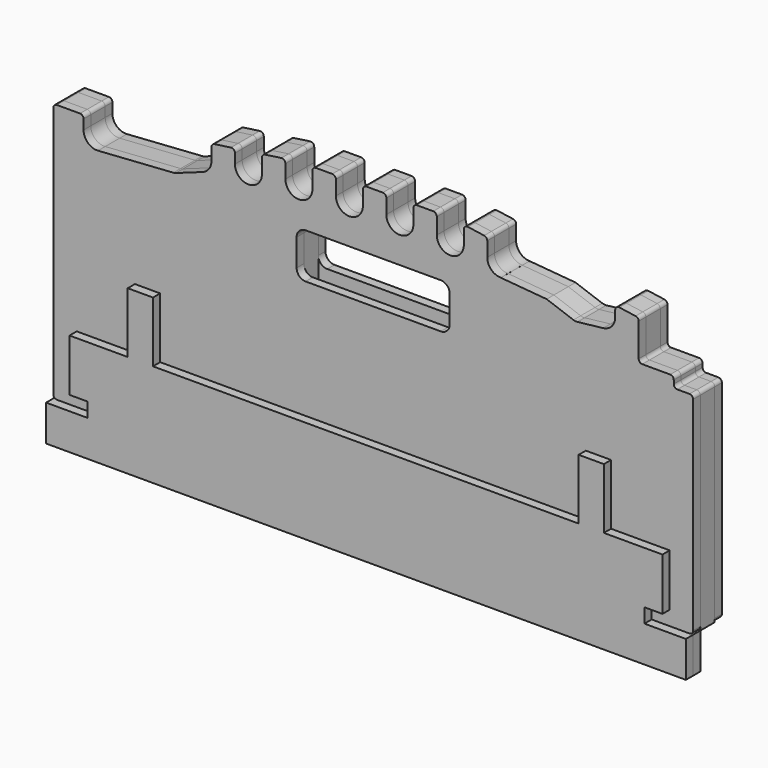
from build123d import *

# Parameters (mm, degrees)
F1_DEPTH  = 12.7
F4_DEPTH  = 12.7
F7_DEPTH  = 6.35
F8_W      = 76.2
F8_H      = 25.4
F9_DEPTH  = 6.35
F13_DEPTH = 25.401
F15_DEPTH = 6.35
F17_DEPTH = 6.35


# Not quite as in the source:
# - ends of sketch curves that miss each other by under 0.0002 mm in the source are joined


with BuildPart() as f1:
    # F0 (on Front) → F1 (new body)
    with BuildSketch(Plane.XZ):
        with BuildLine():
            Line((225.425, -101.6), (225.425, 44.45))
            ThreePointArc((225.425, 44.45), (224.6810512242, 46.2460512242), (222.885, 46.99))
            Line((222.885, 46.99), (214.3453168, 46.99))
            ThreePointArc((214.3453168, 46.99), (212.5492655758, 47.7339487758), (211.8053168, 49.53))
            Line((211.8053168, 49.53), (211.8053168, 52.07))
            ThreePointArc((211.8053168, 52.07), (211.0613680242, 53.8660512242), (209.2653168, 54.61))
            Line((209.2653168, 54.61), (189.611, 54.61))
            ThreePointArc((189.611, 54.61), (187.8149487758, 55.3539487758), (187.071, 57.15))
            Line((187.071, 57.15), (187.071, 80.4293794))
            ThreePointArc((187.071, 80.4293794), (186.4498765809, 82.0935646863), (184.8902813644, 82.9438409529))
            Line((184.8902813644, 82.9438409529), (173.460283, 84.577047))
            ThreePointArc((173.460283, 84.577047), (171.4368160708, 83.9814771579), (170.561, 82.0625994))
            Line((170.561, 82.0625994), (170.561, 77.5154152))
            ThreePointArc((170.561, 77.5154152), (168.1421522313, 71.1728427356), (162.1141285111, 68.0516282247))
            Line((162.1141285111, 68.0516282247), (143.9747438, 65.9851614))
            ThreePointArc((143.9747438, 65.9851614), (142.5270090226, 65.9863525007), (141.1171683546, 66.3154143094))
            Line((141.1171683546, 66.3154143094), (122.267726, 73.058401))
            ThreePointArc((122.267726, 73.058401), (117.6886874549, 76.5419782296), (115.951, 82.0268108))
            Line((115.951, 82.0268108), (115.951, 90.5915638))
            ThreePointArc((115.951, 90.5915638), (115.3298765809, 92.2557490863), (113.7702813644, 93.1060253529))
            Line((113.7702813644, 93.1060253529), (102.340283, 94.7392314))
            ThreePointArc((102.340283, 94.7392314), (100.3168160708, 94.1436615579), (99.441, 92.2247838))
            Line((99.441, 92.2247838), (99.441, 85.3985084))
            ThreePointArc((99.441, 85.3985084), (89.916, 75.8735084), (80.391, 85.3985084))
            Line((80.391, 85.3985084), (80.391, 95.6726814))
            ThreePointArc((80.391, 95.6726814), (79.7698777579, 97.3368653292), (78.2102849211, 98.1871424447))
            Line((78.2102849211, 98.1871424447), (66.780283, 99.820349))
            ThreePointArc((66.780283, 99.820349), (64.7568147137, 99.2247525809), (63.881, 97.305876))
            Line((63.881, 97.305876), (63.881, 87.6407188))
            ThreePointArc((63.881, 87.6407188), (54.356, 78.1157188), (44.831, 87.6407188))
            Line((44.831, 87.6407188), (44.831, 99.06))
            ThreePointArc((44.831, 99.06), (44.0870512242, 100.8560512242), (42.291, 101.6))
            Line((42.291, 101.6), (30.861, 101.6))
            ThreePointArc((30.861, 101.6), (29.0649487758, 100.8560512242), (28.321, 99.06))
            Line((28.321, 99.06), (28.321, 88.7601476))
            ThreePointArc((28.321, 88.7601476), (18.796, 79.2351476), (9.271, 88.7601476))
            Line((9.271, 88.7601476), (9.271, 99.06))
            ThreePointArc((9.271, 99.06), (8.5270512242, 100.8560512242), (6.731, 101.6))
            Line((6.731, 101.6), (-4.699, 101.6))
            ThreePointArc((-4.699, 101.6), (-6.4950512242, 100.8560512242), (-7.239, 99.06))
            Line((-7.239, 99.06), (-7.239, 88.7601476))
            ThreePointArc((-7.239, 88.7601476), (-16.764, 79.2351476), (-26.289, 88.7601476))
            Line((-26.289, 88.7601476), (-26.289, 99.06))
            ThreePointArc((-26.289, 99.06), (-27.0329487758, 100.8560512242), (-28.829, 101.6))
            Line((-28.829, 101.6), (-40.259, 101.6))
            ThreePointArc((-40.259, 101.6), (-42.0550512242, 100.8560512242), (-42.799, 99.06))
            Line((-42.799, 99.06), (-42.799, 87.6407188))
            ThreePointArc((-42.799, 87.6407188), (-52.324, 78.1157188), (-61.849, 87.6407188))
            Line((-61.849, 87.6407188), (-61.849, 97.306257))
            ThreePointArc((-61.849, 97.306257), (-62.7247862201, 99.2251088689), (-64.7482066888, 99.8207292219))
            Line((-64.7482066888, 99.8207292219), (-76.1782068, 98.187891))
            ThreePointArc((-76.1782068, 98.187891), (-77.7378518689, 97.3376317799), (-78.359, 95.673418))
            Line((-78.359, 95.673418), (-78.359, 85.3985084))
            ThreePointArc((-78.359, 85.3985084), (-87.884, 75.8735084), (-97.409, 85.3985084))
            Line((-97.409, 85.3985084), (-97.409, 92.226257))
            ThreePointArc((-97.409, 92.226257), (-98.2847862201, 94.1451088689), (-100.3082066888, 94.7407292219))
            Line((-100.3082066888, 94.7407292219), (-111.7382068, 93.107891))
            ThreePointArc((-111.7382068, 93.107891), (-113.2978518689, 92.2576317799), (-113.919, 90.593418))
            Line((-113.919, 90.593418), (-113.919, 82.0268108))
            ThreePointArc((-113.919, 82.0268108), (-115.6566874549, 76.5419782296), (-120.2357219581, 73.0583897012))
            Line((-120.2357219581, 73.0583897012), (-139.0851676, 66.3154122))
            ThreePointArc((-139.0851676, 66.3154122), (-139.9269299643, 66.0782520994), (-140.7932934765, 65.9589927767))
            Line((-140.7932934765, 65.9589927767), (-193.917951, 62.3473988))
            ThreePointArc((-193.917951, 62.3473988), (-201.0667686949, 64.8905951339), (-204.089, 71.8504532))
            Line((-204.089, 71.8504532), (-204.089, 78.74))
            ThreePointArc((-204.089, 78.74), (-204.8329487758, 80.5360512242), (-206.629, 81.28))
            Line((-206.629, 81.28), (-222.885, 81.28))
            ThreePointArc((-222.885, 81.28), (-224.6810512242, 80.5360512242), (-225.425, 78.74))
            Line((-225.425, 78.74), (-225.425, -101.6))
            Line((-225.425, -101.6), (-193.675, -101.6))
            Line((-193.675, -101.6), (-193.675, -88.9))
            Line((-193.675, -88.9), (-206.375, -88.9))
            Line((-206.375, -88.9), (-206.375, -57.15))
            Line((-206.375, -57.15), (-165.354, -57.15))
            Line((-165.354, -57.15), (-165.354, -14.478))
            Line((-165.354, -14.478), (-152.4, -14.478))
            Line((-152.4, -14.478), (-152.4, -57.15))
            Line((-152.4, -57.15), (152.4, -57.15))
            Line((152.4, -57.15), (152.4, -14.478))
            Line((152.4, -14.478), (165.354, -14.478))
            Line((165.354, -14.478), (165.354, -57.15))
            Line((165.354, -57.15), (206.375, -57.15))
            Line((206.375, -57.15), (206.375, -88.9))
            Line((206.375, -88.9), (193.675, -88.9))
            Line((193.675, -88.9), (193.675, -101.6))
            Line((193.675, -101.6), (225.425, -101.6))
        make_face()
        with BuildLine():
            ThreePointArc((53.9455106, 16.090138), (52.0856386605, 11.6000099395), (47.5955106, 9.740138))
            Line((47.5955106, 9.740138), (-47.5955106, 9.740138))
            ThreePointArc((-47.5955106, 9.740138), (-52.0856386605, 11.6000099395), (-53.9455106, 16.090138))
            Line((-53.9455106, 16.090138), (-53.9455106, 54.190138))
            ThreePointArc((-53.9455106, 54.190138), (-52.0856386605, 58.6802660605), (-47.5955106, 60.540138))
            Line((-47.5955106, 60.540138), (47.5955106, 60.540138))
            ThreePointArc((47.5955106, 60.540138), (52.0856386605, 58.6802660605), (53.9455106, 54.190138))
            Line((53.9455106, 54.190138), (53.9455106, 16.090138))
        make_face(mode=Mode.SUBTRACT)
    extrude(amount=F1_DEPTH)


with BuildPart() as f4:
    # F3 (on offset) → F4 (new body)
    with BuildSketch(Plane(origin=(0, 0, 0), x_dir=(-1, 0, 0), z_dir=(0, 1, 0))):
        Polygon((203.2, -69.85), (-203.2, -69.85), (-203.2, -88.9), (-190.5, -88.9), (-190.5, -114.3), (190.5, -114.3), (190.5, -88.9), (203.2, -88.9), align=None)
    extrude(amount=-F4_DEPTH)


with BuildPart() as f7:
    # F6 (on offset) → F7 (new body)
    with BuildSketch(Plane(origin=(0, 0, 0), x_dir=(-1, 0, 0), z_dir=(0, 1, 0))):
        with BuildLine():
            ThreePointArc((-222.885, 46.99), (-224.6810512242, 46.2460512242), (-225.425, 44.45))
            Line((-225.425, 44.45), (-225.425, -99.06))
            ThreePointArc((-225.425, -99.06), (-224.6810512242, -100.8560512242), (-222.885, -101.6))
            Line((-222.885, -101.6), (222.885, -101.6))
            ThreePointArc((222.885, -101.6), (224.6810512242, -100.8560512242), (225.425, -99.06))
            Line((225.425, -99.06), (225.425, 78.74))
            ThreePointArc((225.425, 78.74), (224.6810512242, 80.5360512242), (222.885, 81.28))
            Line((222.885, 81.28), (206.629, 81.28))
            ThreePointArc((206.629, 81.28), (204.8329487758, 80.5360512242), (204.089, 78.74))
            Line((204.089, 78.74), (204.089, 71.8504532))
            ThreePointArc((204.089, 71.8504532), (201.0667686949, 64.8905951339), (193.9179502781, 62.3473881809))
            Line((193.9179502781, 62.3473881809), (140.7933176, 65.958974))
            ThreePointArc((140.7933176, 65.958974), (139.9269423678, 66.0782495112), (139.0851683546, 66.3154143094))
            Line((139.0851683546, 66.3154143094), (120.2357514, 73.058401))
            ThreePointArc((120.2357514, 73.058401), (115.6566943407, 76.5419684532), (113.919, 82.0268108))
            Line((113.919, 82.0268108), (113.919, 90.593418))
            ThreePointArc((113.919, 90.593418), (113.2978601063, 92.257622282), (111.7382315808, 93.1078866658))
            Line((111.7382315808, 93.1078866658), (100.3082322, 94.74073))
            ThreePointArc((100.3082322, 94.74073), (98.284795718, 94.1451171063), (97.409, 92.226257))
            Line((97.409, 92.226257), (97.409, 85.3985084))
            ThreePointArc((97.409, 85.3985084), (87.884, 75.8735084), (78.359, 85.3985084))
            Line((78.359, 85.3985084), (78.359, 95.673418))
            ThreePointArc((78.359, 95.673418), (77.7378601063, 97.337622282), (76.1782315808, 98.1878866658))
            Line((76.1782315808, 98.1878866658), (64.7482322, 99.82073))
            ThreePointArc((64.7482322, 99.82073), (62.724795718, 99.2251171063), (61.849, 97.306257))
            Line((61.849, 97.306257), (61.849, 87.6407188))
            ThreePointArc((61.849, 87.6407188), (52.324, 78.1157188), (42.799, 87.6407188))
            Line((42.799, 87.6407188), (42.799, 99.06))
            ThreePointArc((42.799, 99.06), (42.0550512242, 100.8560512242), (40.259, 101.6))
            Line((40.259, 101.6), (28.829, 101.6))
            ThreePointArc((28.829, 101.6), (27.0329487758, 100.8560512242), (26.289, 99.06))
            Line((26.289, 99.06), (26.289, 88.7601476))
            ThreePointArc((26.289, 88.7601476), (16.764, 79.2351476), (7.239, 88.7601476))
            Line((7.239, 88.7601476), (7.239, 99.06))
            ThreePointArc((7.239, 99.06), (6.4950512242, 100.8560512242), (4.699, 101.6))
            Line((4.699, 101.6), (-6.731, 101.6))
            ThreePointArc((-6.731, 101.6), (-8.5270512242, 100.8560512242), (-9.271, 99.06))
            Line((-9.271, 99.06), (-9.271, 88.7601476))
            ThreePointArc((-9.271, 88.7601476), (-18.796, 79.2351476), (-28.321, 88.7601476))
            Line((-28.321, 88.7601476), (-28.321, 99.06))
            ThreePointArc((-28.321, 99.06), (-29.0649487758, 100.8560512242), (-30.861, 101.6))
            Line((-30.861, 101.6), (-42.291, 101.6))
            ThreePointArc((-42.291, 101.6), (-44.0870512242, 100.8560512242), (-44.831, 99.06))
            Line((-44.831, 99.06), (-44.831, 87.6407188))
            ThreePointArc((-44.831, 87.6407188), (-54.356, 78.1157188), (-63.881, 87.6407188))
            Line((-63.881, 87.6407188), (-63.881, 97.305876))
            ThreePointArc((-63.881, 97.305876), (-64.7568147137, 99.2247525809), (-66.7802813644, 99.8203375529))
            Line((-66.7802813644, 99.8203375529), (-78.210283, 98.187129))
            ThreePointArc((-78.210283, 98.187129), (-79.7698777579, 97.3368653292), (-80.391, 95.6726814))
            Line((-80.391, 95.6726814), (-80.391, 85.3985084))
            ThreePointArc((-80.391, 85.3985084), (-89.916, 75.8735084), (-99.441, 85.3985084))
            Line((-99.441, 85.3985084), (-99.441, 92.2247838))
            ThreePointArc((-99.441, 92.2247838), (-100.3168160708, 94.1436615579), (-102.3402849211, 94.7392448447))
            Line((-102.3402849211, 94.7392448447), (-113.770283, 93.1060368))
            ThreePointArc((-113.770283, 93.1060368), (-115.3298765809, 92.2557490863), (-115.951, 90.5915638))
            Line((-115.951, 90.5915638), (-115.951, 82.0268108))
            ThreePointArc((-115.951, 82.0268108), (-117.6886874549, 76.5419782296), (-122.2677219581, 73.0583897012))
            Line((-122.2677219581, 73.0583897012), (-141.1171422, 66.3154122))
            ThreePointArc((-141.1171422, 66.3154122), (-142.5269971438, 65.9863538735), (-143.9747420782, 65.985176514))
            Line((-143.9747420782, 65.985176514), (-162.114103, 68.0516292))
            ThreePointArc((-162.114103, 68.0516292), (-168.1421438289, 71.1728333216), (-170.561, 77.5154152))
            Line((-170.561, 77.5154152), (-170.561, 82.0625994))
            ThreePointArc((-170.561, 82.0625994), (-171.4368160708, 83.9814771579), (-173.4602849211, 84.5770604447))
            Line((-173.4602849211, 84.5770604447), (-184.890283, 82.9438524))
            ThreePointArc((-184.890283, 82.9438524), (-186.4498765809, 82.0935646863), (-187.071, 80.4293794))
            Line((-187.071, 80.4293794), (-187.071, 57.15))
            ThreePointArc((-187.071, 57.15), (-187.8149487758, 55.3539487758), (-189.611, 54.61))
            Line((-189.611, 54.61), (-209.2652914, 54.61))
            ThreePointArc((-209.2652914, 54.61), (-211.0613426242, 53.8660512242), (-211.8052914, 52.07))
            Line((-211.8052914, 52.07), (-211.8052914, 49.53))
            ThreePointArc((-211.8052914, 49.53), (-212.5492401758, 47.7339487758), (-214.3452914, 46.99))
            Line((-214.3452914, 46.99), (-222.885, 46.99))
        make_face()
        with BuildLine():
            Line((47.595536, 28.7862264), (-47.5955106, 28.7862264))
            ThreePointArc((-47.5955106, 28.7862264), (-52.0856386605, 30.6460983395), (-53.9455106, 35.1362264))
            Line((-53.9455106, 35.1362264), (-53.9455106, 54.1862264))
            ThreePointArc((-53.9455106, 54.1862264), (-52.0856386605, 58.6763544605), (-47.5955106, 60.5362264))
            Line((-47.5955106, 60.5362264), (47.595536, 60.5362264))
            ThreePointArc((47.595536, 60.5362264), (52.0856640605, 58.6763544605), (53.945536, 54.1862264))
            Line((53.945536, 54.1862264), (53.945536, 35.1362264))
            ThreePointArc((53.945536, 35.1362264), (52.0856640605, 30.6460983395), (47.595536, 28.7862264))
        make_face(mode=Mode.SUBTRACT)
    extrude(amount=F7_DEPTH)

    # F8 (on face) → F9 (cut)
    with BuildSketch(Plane(origin=(0, 6.35, 0), x_dir=(-1, 0, 0), z_dir=(0, 1, 0))):
        with Locations((-1.27, -88.9)):
            Rectangle(F8_W, F8_H)
    extrude(amount=-F9_DEPTH, mode=Mode.SUBTRACT)


with BuildPart() as f10_1:
    # F10: instance of F7
    add(f7.part.mirror(Plane(origin=(-1.6757750032, -6.35, 6.749495993), x_dir=(1, 0, 0), z_dir=(0, 1, 0))))


with BuildPart() as f13_tool:
    # F12 (on offset) → F13 (new body, through all)
    with BuildSketch(Plane.XZ.offset(19.05)):
        Polygon((89.916, 75.8384061145), (122.2677219581, 73.0583897012), (119.4564439139, 93.1060368), (99.441, 97.305876), align=None)
    extrude(amount=-F13_DEPTH)


with BuildPart() as f1_1:
    add(f1.part)

    # F13: cut by f13_tool
    add(f13_tool.part, mode=Mode.SUBTRACT)


with BuildPart() as f7_1:
    add(f7.part)

    # F13: cut by f13_tool
    add(f13_tool.part, mode=Mode.SUBTRACT)


with BuildPart() as f10_1_1:
    add(f10_1.part)

    # F13: cut by f13_tool
    add(f13_tool.part, mode=Mode.SUBTRACT)


with BuildPart() as f15:
    # F14 (on face) → F15 (new body)
    with BuildSketch(Plane.XZ.offset(12.7)):
        Polygon((-36.83, -101.6), (-225.425, -101.6), (-225.425, -127), (225.425, -127), (225.425, -101.6), (39.37, -101.6), (39.37, -76.2), (-36.83, -76.2), align=None)
    extrude(amount=F15_DEPTH)


with BuildPart() as f17:
    # F16 (on face) → F17 (new body)
    with BuildSketch(Plane.XZ.offset(19.05)):
        Polygon((-196.215, -101.6), (-225.425, -101.6), (-225.425, -127), (225.425, -127), (225.425, -101.6), (196.215, -101.6), (196.215, -91.44), (208.915, -91.44), (208.915, -54.61), (167.64, -54.61), (167.64, -11.938), (149.86, -11.938), (149.86, -54.61), (-150.114, -54.61), (-150.114, -11.938), (-167.894, -11.938), (-167.894, -54.61), (-208.915, -54.61), (-208.915, -91.44), (-196.215, -91.44), align=None)
    extrude(amount=F17_DEPTH)


solid = Compound([f4.part, f1_1.part, f7_1.part, f10_1_1.part, f15.part, f17.part])
